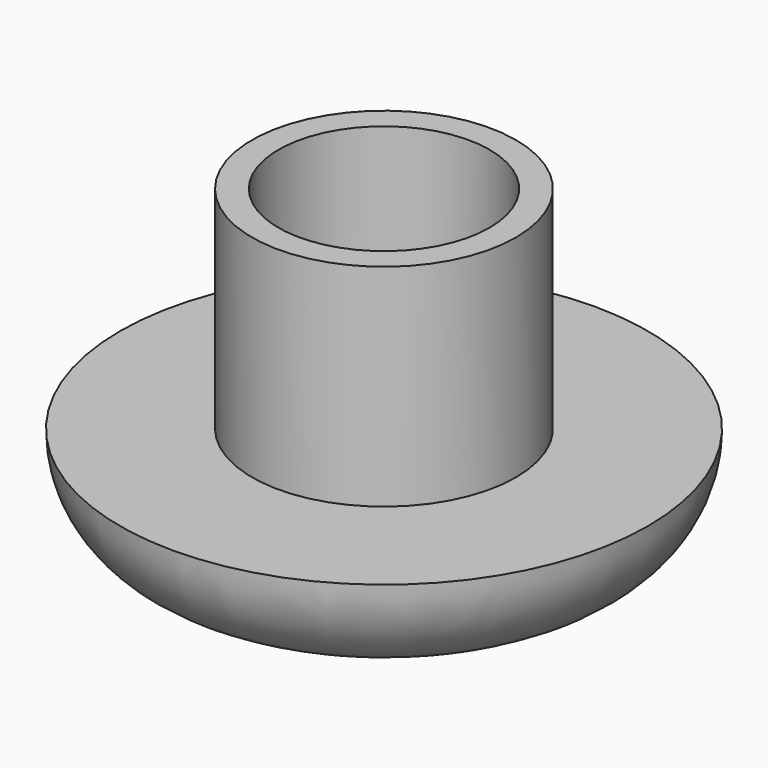
from build123d import *

# Parameters (mm, degrees)
F0_R     = 5
F0_R_2   = 2
F2_DEPTH = 2
F3_R     = 2.5
F3_R_2   = 2
F4_DEPTH = 4
F5_R     = 1.99999


# Not quite as in the source:
# - a fillet or chamfer is up to 0.001 mm smaller than in the source, because OpenCascade refuses the exact size


with BuildPart() as f2:
    # F0 (on Top) → F2 (new body)
    with BuildSketch(Plane.XY):
        Circle(F0_R)
        Circle(F0_R_2, mode=Mode.SUBTRACT)
    extrude(amount=F2_DEPTH)

    # F3 (on face) → F4 (join)
    with BuildSketch(Plane.XY.offset(2)):
        Circle(F3_R)
        Circle(F3_R_2, mode=Mode.SUBTRACT)
    extrude(amount=F4_DEPTH)

    # F5 (radius 2 in the source; OpenCascade refuses exactly that, so slightly less here)
    f5_edges = [f2.edges().sort_by_distance(p)[0] for p in [
        (-5, 0, 0),
    ]]
    fillet(f5_edges, radius=F5_R)


solid = f2.part
